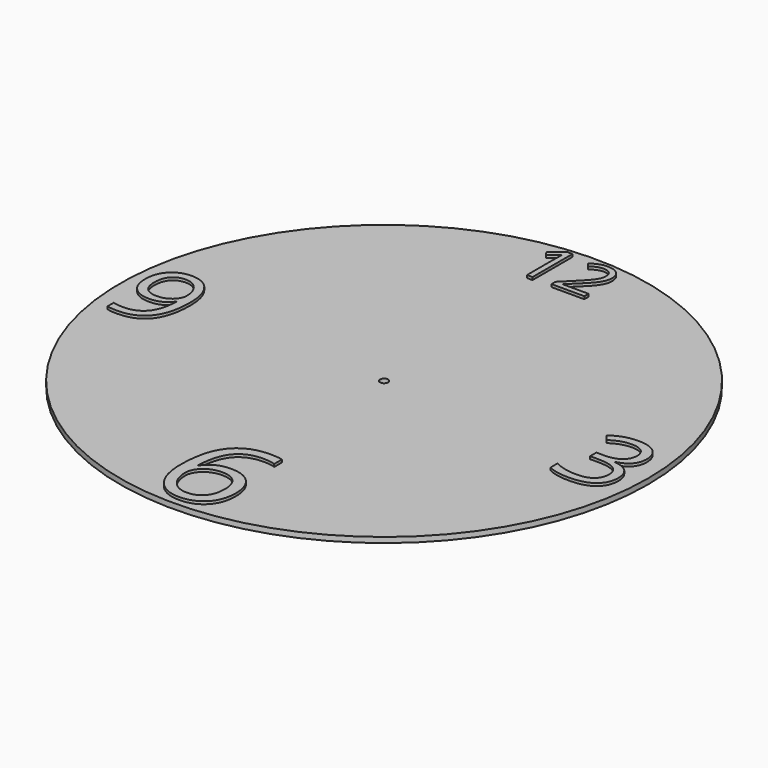
from build123d import *

# Parameters (mm, degrees)
F0_R           = 98
F1_DEPTH       = 2
F2_TEXT_SIZE   = 25.9810554804
F2_TEXT_SIZE_2 = 51.0366826156
F2_TEXT_SIZE_3 = 41.6666666667
F3_DEPTH       = 1
F4_R           = 1.5
F5_DEPTH       = 4


# Not quite as in the source:
# - Text() gives the source's letters only with a copy of the font that has no kerning and outlines rounded to 1/6400 em; it was checked with that copy


with BuildPart() as f1:
    # F0 (on Top) → F1 (new body)
    with BuildSketch(Plane.XY):
        Circle(F0_R)
    extrude(amount=F1_DEPTH)

    # F2 (on face) → F3 (join)
    with BuildSketch(Plane.XY.offset(2)):
        with Locations((-15, 76.2936400541)):
            Text('12', F2_TEXT_SIZE, font='Open Sans', text_align=(TextAlign.LEFT, TextAlign.BOTTOM))
        with Locations((-15, -95)):
            Text('6', F2_TEXT_SIZE_2, font='Open Sans', text_align=(TextAlign.LEFT, TextAlign.BOTTOM))
        with Locations((70.91796875, -15)):
            Text('3', F2_TEXT_SIZE_3, font='Open Sans', text_align=(TextAlign.LEFT, TextAlign.BOTTOM))
        with Locations((-95, -15)):
            Text('9', F2_TEXT_SIZE_3, font='Open Sans', text_align=(TextAlign.LEFT, TextAlign.BOTTOM))
    extrude(amount=F3_DEPTH)

    # F4 (on face) → F5 (cut)
    with BuildSketch(Plane.XY.offset(2)):
        Circle(F4_R)
    extrude(amount=-F5_DEPTH, mode=Mode.SUBTRACT)


solid = f1.part
